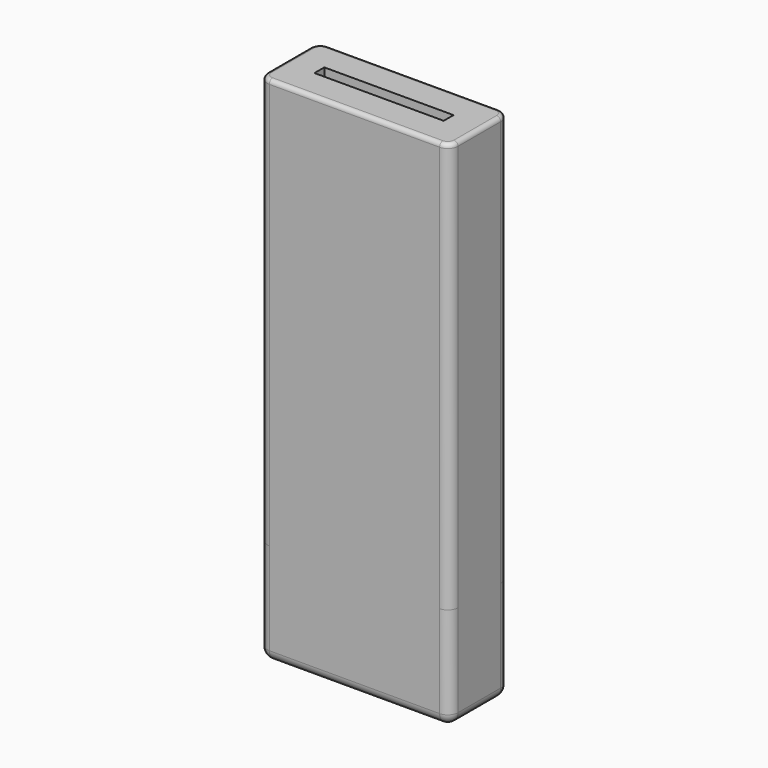
from build123d import *

# Parameters (mm, degrees)
F0_W     = 23.622
F0_H     = 9.144
F1_DEPTH = 12.7
F2_R     = 1.27
F3_W     = 16.002
F3_H     = 1.524
F4_DEPTH = 50.8
F5_R     = 0.508


with BuildPart() as f1:
    # F0 (on Top) → F1 (new body)
    with BuildSketch(Plane.XY):
        with Locations((-8.5595357362, -22.114415653)):
            Rectangle(F0_W, F0_H)
    extrude(amount=F1_DEPTH)

    # F2
    f2_edges = [f1.edges().sort_by_distance(p)[0] for p in [
        (-8.559536, -26.686416, 0),
        (-20.370536, -22.114416, 0),
        (-8.559536, -17.542416, 0),
        (3.251464, -22.114416, 0),
        (3.251464, -17.542416, 6.35),
        (-20.370536, -17.542416, 6.35),
        (-20.370536, -26.686416, 6.35),
        (3.251464, -26.686416, 6.35),
    ]]
    fillet(f2_edges, radius=F2_R)

    # F3 (on face) → F4 (join)
    with BuildSketch(Plane.XY.offset(12.7)):
        with BuildLine():
            ThreePointArc((3.2514642638, -18.812415653), (2.8794898759, -17.9143900409), (1.9814642638, -17.542415653))
            Line((1.9814642638, -17.542415653), (-19.1005357362, -17.542415653))
            ThreePointArc((-19.1005357362, -17.542415653), (-19.9985613483, -17.9143900409), (-20.3705357362, -18.812415653))
            Line((-20.3705357362, -18.812415653), (-20.3705357362, -25.416415653))
            ThreePointArc((-20.3705357362, -25.416415653), (-19.9985613483, -26.3144412652), (-19.1005357362, -26.686415653))
            Line((-19.1005357362, -26.686415653), (1.9814642638, -26.686415653))
            ThreePointArc((1.9814642638, -26.686415653), (2.8794898759, -26.3144412652), (3.2514642638, -25.416415653))
            Line((3.2514642638, -25.416415653), (3.2514642638, -18.812415653))
        make_face()
        with Locations((-8.5595357362, -22.114415653)):
            Rectangle(F3_W, F3_H, mode=Mode.SUBTRACT)
    extrude(amount=F4_DEPTH)

    # F5
    f5_edges = [f1.edges().sort_by_distance(p)[0] for p in [
        (-8.559536, -17.542416, 63.5),
        (3.251464, -22.114416, 63.5),
        (-8.559536, -26.686416, 63.5),
        (-20.370536, -22.114416, 63.5),
        (2.87949, -26.314441, 63.5),
        (-19.998561, -26.314441, 63.5),
        (-19.998561, -17.91439, 63.5),
        (2.87949, -17.91439, 63.5),
    ]]
    fillet(f5_edges, radius=F5_R)


solid = f1.part
